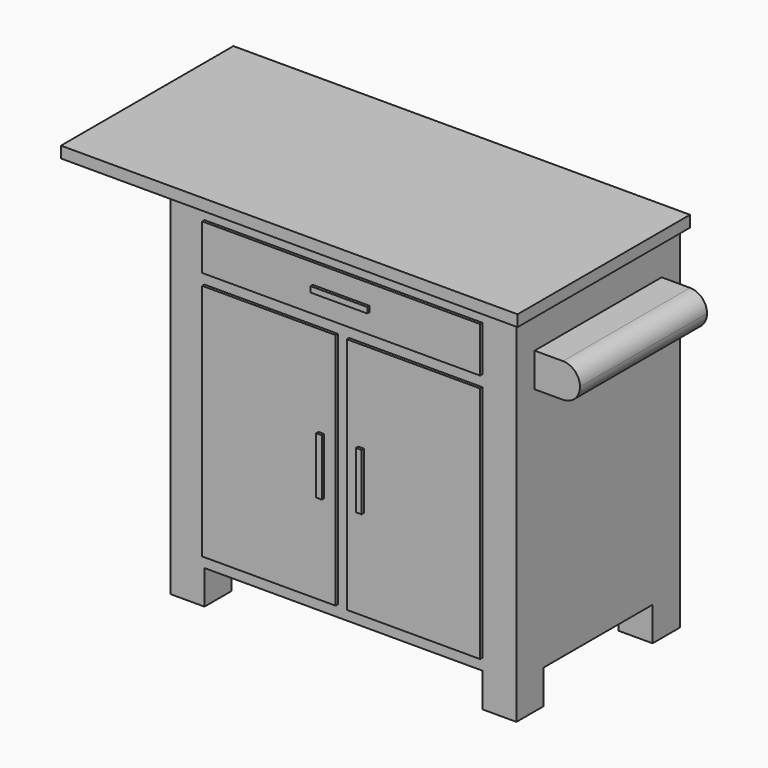
from build123d import *

# Parameters (mm, degrees)
F0_W      = 76.2
F0_H      = 76.2
F1_DEPTH  = 812.8
F2_DEPTH  = 736.6
F0_W_2    = 800.1
F0_H_2    = 482.6
F3_DEPTH  = 25.4
F4_W      = 355.6
F4_H      = 76.2
F5_DEPTH  = 101.6
F6_R      = 38.09999
F7_W      = 298.45
F7_H      = 533.4
F7_W_2    = 12.7
F7_H_2    = 127
F7_W_3    = 622.3
F7_H_3    = 101.6
F7_W_4    = 127
F7_H_4    = 12.7
F8_DEPTH  = 6.35
F9_DEPTH  = 12.7
F10_W     = 222.25
F10_H     = 482.6
F11_DEPTH = 25.4
F12_W     = 622.3
F12_H     = 304.8
F13_DEPTH = 635


# Not quite as in the source:
# - a fillet or chamfer is up to 0.001 mm smaller than in the source, because OpenCascade refuses the exact size


with BuildPart() as f1:
    # F0 (on Top) → F1 (new body)
    with BuildSketch(Plane.XY):
        with Locations((-349.25, 190.5)):
            Rectangle(F0_W, F0_H)
    extrude(amount=-F1_DEPTH)



with BuildPart() as f1b:
    # F0 (on Top) → F1, piece 2 (new body)
    with BuildSketch(Plane.XY):
        with Locations((-349.25, -190.5)):
            Rectangle(F0_W, F0_H)
    extrude(amount=-F1_DEPTH)


with BuildPart() as f1c:
    # F0 (on Top) → F1, piece 3 (new body)
    with BuildSketch(Plane.XY):
        with Locations((349.25, -190.5)):
            Rectangle(F0_W, F0_H)
    extrude(amount=-F1_DEPTH)


with BuildPart() as f1d:
    # F0 (on Top) → F1, piece 4 (new body)
    with BuildSketch(Plane.XY):
        with Locations((349.25, 190.5)):
            Rectangle(F0_W, F0_H)
    extrude(amount=-F1_DEPTH)


with BuildPart() as f1_1:
    add(f1.part)

    add(f1b.part)  # F2 merges F1b

    add(f1c.part)  # F2 merges F1c

    add(f1d.part)  # F2 merges F1d
    # F0 (on Top) → F2 (join)
    with BuildSketch(Plane.XY):
        with Locations((-349.25, 190.5)):
            Rectangle(F0_W, F0_H)
        Polygon((311.15, 152.4), (311.15, 228.6), (-311.15, 228.6), (-311.15, 152.4), (-387.35, 152.4), (-387.35, -152.4), (-311.15, -152.4), (-311.15, -228.6), (311.15, -228.6), (311.15, -152.4), (387.35, -152.4), (387.35, 152.4), align=None)
        with Locations((-349.25, -190.5)):
            Rectangle(F0_W, F0_H)
        with Locations((349.25, -190.5)):
            Rectangle(F0_W, F0_H)
        with Locations((349.25, 190.5)):
            Rectangle(F0_W, F0_H)
    extrude(amount=-F2_DEPTH)

    # F0 (on Top) → F3 (join)
    with BuildSketch(Plane.XY):
        Rectangle(F0_W_2, F0_H_2)
        Polygon((311.15, 228.6), (387.35, 228.6), (387.35, 152.4), (387.35, -152.4), (387.35, -228.6), (311.15, -228.6), (-311.15, -228.6), (-387.35, -228.6), (-387.35, -152.4), (-387.35, 152.4), (-387.35, 228.6), (-311.15, 228.6), align=None, mode=Mode.SUBTRACT)
    extrude(amount=-F3_DEPTH)

    # F4 (on face) → F5 (join)
    with BuildSketch(Plane.YZ.offset(387.35)):
        with Locations((0, -139.7)):
            Rectangle(F4_W, F4_H)
    extrude(amount=F5_DEPTH)

    # F6 (radius 38.1 in the source; OpenCascade refuses exactly that, so slightly less here)
    f6_edges = [f1_1.edges().sort_by_distance(p)[0] for p in [
        (488.95, 0, -101.6),
        (488.95, 0, -177.8),
    ]]
    fillet(f6_edges, radius=F6_R)

    # F7 (on face) → F8 (join)
    with BuildSketch(Plane.XZ.offset(228.6)):
        with Locations((161.925, -444.5)):
            Rectangle(F7_W, F7_H)
        with Locations((44.45, -444.5)):
            Rectangle(F7_W_2, F7_H_2, mode=Mode.SUBTRACT)
        with Locations((-161.925, -444.5)):
            Rectangle(F7_W, F7_H)
        with Locations((-44.45, -444.5)):
            Rectangle(F7_W_2, F7_H_2, mode=Mode.SUBTRACT)
        with Locations((0, -101.6)):
            Rectangle(F7_W_3, F7_H_3)
        with Locations((0, -101.6)):
            Rectangle(F7_W_4, F7_H_4, mode=Mode.SUBTRACT)
        with Locations((0, -101.6)):
            Rectangle(F7_W_4, F7_H_4)
        with Locations((44.45, -444.5)):
            Rectangle(F7_W_2, F7_H_2)
        with Locations((-44.45, -444.5)):
            Rectangle(F7_W_2, F7_H_2)
    extrude(amount=F8_DEPTH)

    # F7 (on face) → F9 (join)
    with BuildSketch(Plane.XZ.offset(228.6)):
        with Locations((0, -101.6)):
            Rectangle(F7_W_4, F7_H_4)
        with Locations((-44.45, -444.5)):
            Rectangle(F7_W_2, F7_H_2)
        with Locations((44.45, -444.5)):
            Rectangle(F7_W_2, F7_H_2)
    extrude(amount=F9_DEPTH)

    # F10 (on face) → F11 (join, through all)
    with BuildSketch(Plane.XY):
        with Locations((-511.175, 0)):
            Rectangle(F10_W, F10_H)
    extrude(amount=-F11_DEPTH)

    # F12 (on face) → F13 (cut)
    with BuildSketch(Plane(origin=(0, 0, -736.6), x_dir=(1, 0, 0), z_dir=(0, 0, -1))):
        Rectangle(F12_W, F12_H)
    extrude(amount=-F13_DEPTH, mode=Mode.SUBTRACT)


solid = f1_1.part
